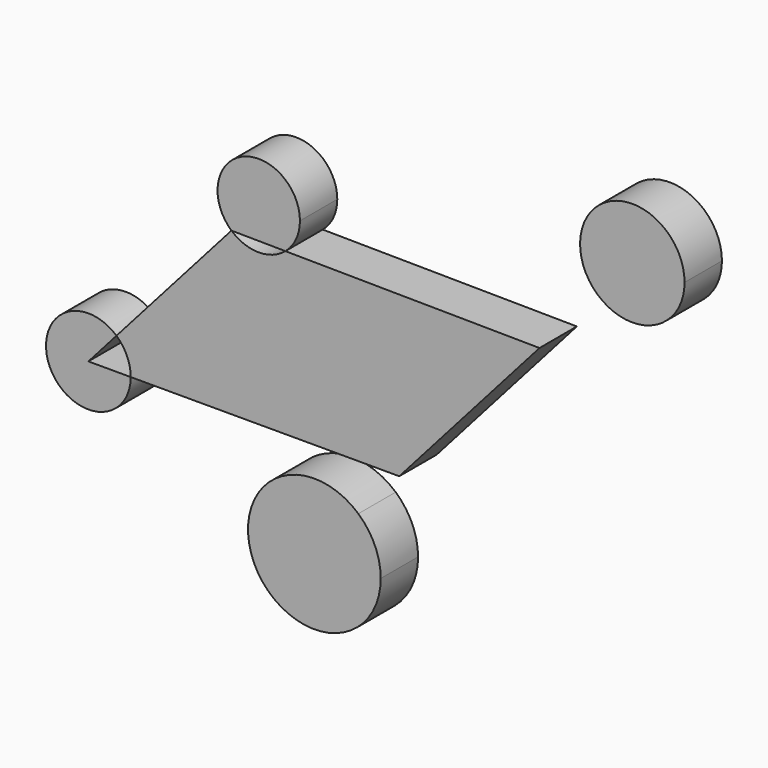
from build123d import *

# Parameters (mm, degrees)
F1_DEPTH = 25.4


with BuildPart() as f1:
    # F0 (on Front) → F1 (new body)
    with BuildSketch(Plane.XZ):
        with BuildLine():
            Line((-106.9061532036, -28.9377868176), (-129.9478113651, -28.9377868176))
            Line((-129.9478113651, -28.9377868176), (-114.6803066145, -11.6802867227))
            ThreePointArc((-114.6803066145, -11.6802867227), (-150.9562220175, -38.4016492793), (-106.9061532036, -28.9377868176))
        make_face()
    extrude(amount=F1_DEPTH)


with BuildPart() as f1b:
    # F0 (on Front) → F1, piece 2 (new body)
    with BuildSketch(Plane.XZ):
        with BuildLine():
            ThreePointArc((194.3457171495, 114.3488910523), (154.2573533816, 140.2581148478), (147.0998454016, 93.0655850704))
            ThreePointArc((147.0998454016, 93.0655850704), (177.6005119431, 88.4396672568), (194.3457171495, 114.3488910523))
        make_face()
    extrude(amount=F1_DEPTH)


with BuildPart() as f1c:
    # F0 (on Front) → F1, piece 3 (new body)
    with BuildSketch(Plane.XZ):
        with BuildLine():
            ThreePointArc((29.0746289373, -81.1474440853), (25.8891745461, -66.3205712619), (16.8949946285, -54.1104113526))
            ThreePointArc((16.8949946285, -54.1104113526), (-39.9378668388, -95.9743169088), (29.0746289373, -81.1474440853))
        make_face()
    extrude(amount=F1_DEPTH)


with BuildPart() as f1d:
    # F0 (on Front) → F1, piece 4 (new body)
    with BuildSketch(Plane.XZ):
        with BuildLine():
            Line((-52.1326156147, 59.019988207), (-114.6803066145, -11.6802867227))
            ThreePointArc((-114.6803066145, -11.6802867227), (-108.9394007128, -19.4739243558), (-106.9061532036, -28.9377868176))
            Line((-106.9061532036, -28.9377868176), (39.1649156809, -28.9377868176))
            Line((39.1649156809, -28.9377868176), (115.4399755566, 57.2791081198))
            Line((115.4399755566, 57.2791081198), (-22.7859247841, 58.7151109634))
            ThreePointArc((-22.7859247841, 58.7151109634), (-37.5161185324, 53.3954768475), (-52.1326156147, 59.019988207))
        make_face()
    extrude(amount=F1_DEPTH)


with BuildPart() as f1e:
    # F0 (on Front) → F1, piece 5 (new body)
    with BuildSketch(Plane.XZ):
        with BuildLine():
            ThreePointArc((-14.8728026772, 75.8047774434), (-46.4879444812, 96.2377337264), (-52.1326156147, 59.019988207))
            Line((-52.1326156147, 59.019988207), (-22.7859247841, 58.7151109634))
            ThreePointArc((-22.7859247841, 58.7151109634), (-16.9470788229, 66.3883794873), (-14.8728026772, 75.8047774434))
        make_face()
    extrude(amount=F1_DEPTH)


solid = Compound([f1.part, f1b.part, f1c.part, f1d.part, f1e.part])
